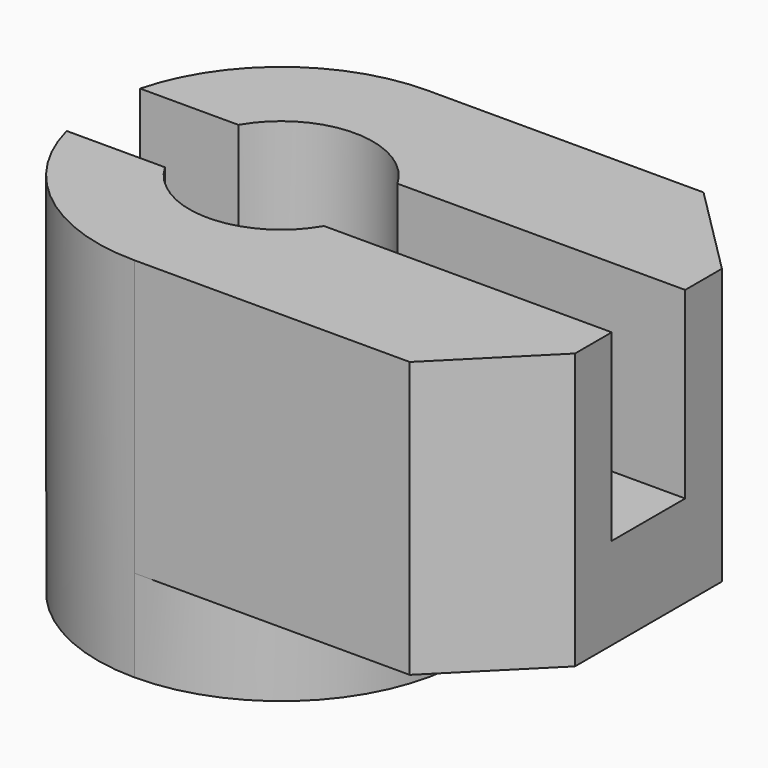
from build123d import *
from build123d import SkipClean  # not in build123d's __all__

# Parameters (mm, degrees)
F0_R     = 5
F1_DEPTH = 20
F2_DEPTH = 20
F3_W     = 5
F3_H     = 10
F4_DEPTH = 30
F5_DEPTH = 5


with BuildPart() as f1:
    # F0 (on Top) → F1 (new body)
    with BuildSketch(Plane.XY):
        with BuildLine():
            ThreePointArc((0, -10), (7.0710678119, -7.0710678119), (10, 0))
            ThreePointArc((10, 0), (7.0710678119, 7.0710678119), (0, 10))
            ThreePointArc((0, 10), (-10, 0), (0, -10))
        make_face()
        Circle(F0_R, mode=Mode.SUBTRACT)
    extrude(amount=F1_DEPTH)

    # F0 (on Top) → F2 (join)
    with BuildSketch(Plane.XY):
        with BuildLine():
            ThreePointArc((0, 10), (7.0710678119, 7.0710678119), (10, 0))
            ThreePointArc((10, 0), (7.0710678119, -7.0710678119), (0, -10))
            Line((0, -10), (15, -10))
            Line((15, -10), (20, -5))
            Line((20, -5), (20, 5))
            Line((20, 5), (15, 10))
            Line((15, 10), (0, 10))
        make_face()
    extrude(amount=F2_DEPTH)

    # F3 (on face) → F4 (cut)
    with BuildSketch(Plane.YZ.offset(20)):
        with Locations((0, 15)):
            Rectangle(F3_W, F3_H)
    extrude(amount=-F4_DEPTH, mode=Mode.SUBTRACT)

    # F0 (on Top) → F5 (cut)
    with BuildSketch(Plane.XY):
        with BuildLine():
            ThreePointArc((0, 10), (7.0710678119, 7.0710678119), (10, 0))
            ThreePointArc((10, 0), (7.0710678119, -7.0710678119), (0, -10))
            Line((0, -10), (15, -10))
            Line((15, -10), (20, -5))
            Line((20, -5), (20, 5))
            Line((20, 5), (15, 10))
            Line((15, 10), (0, 10))
        make_face()
    with SkipClean():  # cleaning this boolean's faces spoils the solid; the shape is the same uncleaned
        extrude(amount=F5_DEPTH, mode=Mode.SUBTRACT)


solid = f1.part
